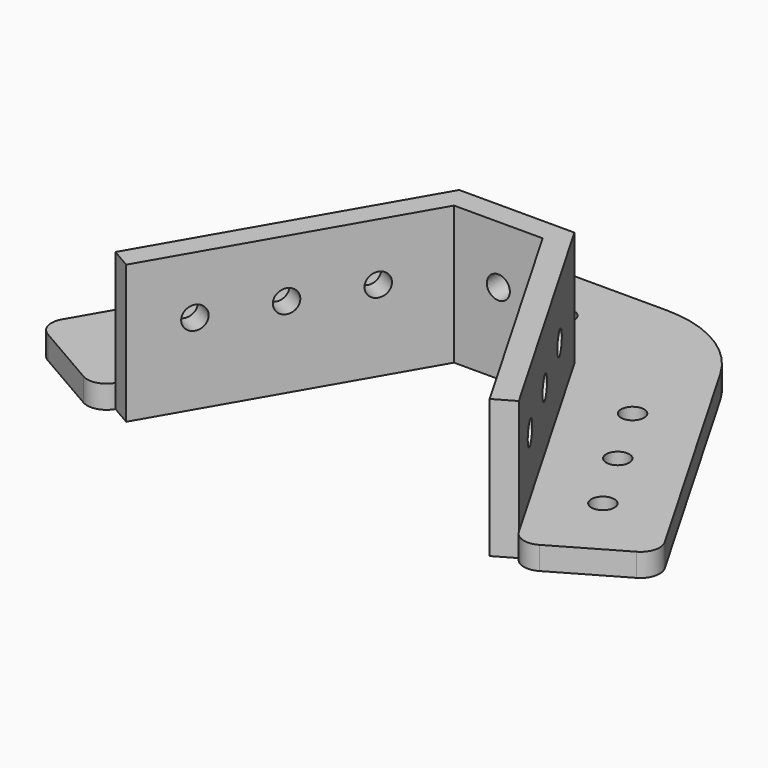
from build123d import *

# Parameters (mm, degrees)
F0_R          = 3
F1_DEPTH      = 6
F2_R          = 5
F3_R          = 5
F4_R          = 5
F5_R          = 5
F7_DEPTH      = 30
F7_DEPTH_BACK = 6
F8_R          = 3
F9_DEPTH      = 76.5570802573
F10_R         = 3
F11_DEPTH     = 36.0010005965


# Not quite as in the source:
# - a pattern or mirror of a feature is missing from the dataset's text; its kind, count and spacing are read off the source's solid


with BuildPart() as f1:
    # F0 (on Top) → F1 (new body)
    with BuildSketch(Plane.XY):
        with BuildLine():
            Line((15, 36.5101838864), (-15, 36.5101838864))
            ThreePointArc((-15, 36.5101838864), (-30, 32.490946), (-40.9807621135, 21.5101838864))
            Line((-40.9807621135, 21.5101838864), (-80.9807621135, -47.7718484163))
            Line((-80.9807621135, -47.7718484163), (-55, -62.7718484163))
            Line((-55, -62.7718484163), (-15, 6.5101838864))
            Line((-15, 6.5101838864), (15, 6.5101838864))
            Line((15, 6.5101838864), (55, -62.7718484163))
            Line((55, -62.7718484163), (80.9807621135, -47.7718484163))
            Line((80.9807621135, -47.7718484163), (40.9807621135, 21.5101838864))
            ThreePointArc((40.9807621135, 21.5101838864), (30, 32.490946), (15, 36.5101838864))
        make_face()
        with Locations((-57.9903810568, -37.9513403406)):
            Circle(F0_R, mode=Mode.SUBTRACT)
        with Locations((-47.9903810568, -20.6308322649)):
            Circle(F0_R, mode=Mode.SUBTRACT)
        with Locations((57.9903810568, -37.9513403406)):
            Circle(F0_R, mode=Mode.SUBTRACT)
        with Locations((47.9903810568, -20.6308322649)):
            Circle(F0_R, mode=Mode.SUBTRACT)
        with Locations((-37.9903810568, -3.3103241892)):
            Circle(F0_R, mode=Mode.SUBTRACT)
        with Locations((37.9903810568, -3.3103241892)):
            Circle(F0_R, mode=Mode.SUBTRACT)
        with Locations((0, 21.5101838864)):
            Circle(F0_R, mode=Mode.SUBTRACT)
    extrude(amount=F1_DEPTH)

    # F2
    f2_edges = [f1.edges().sort_by_distance(p)[0] for p in [
        (80.980762, -47.771848, 3),
    ]]
    fillet(f2_edges, radius=F2_R)

    # F3
    f3_edges = [f1.edges().sort_by_distance(p)[0] for p in [
        (55, -62.771848, 3),
    ]]
    fillet(f3_edges, radius=F3_R)

    # F4
    f4_edges = [f1.edges().sort_by_distance(p)[0] for p in [
        (-55, -62.771848, 3),
    ]]
    fillet(f4_edges, radius=F4_R)

    # F5
    f5_edges = [f1.edges().sort_by_distance(p)[0] for p in [
        (-80.980762, -47.771848, 3),
    ]]
    fillet(f5_edges, radius=F5_R)


with BuildPart() as f7:
    # F6 (on face) → F7 (new body, two sides)
    with BuildSketch(Plane.XY.offset(6)) as f7_sk:
        Polygon((52.5, -58.4417213974), (15, 6.5101838864), (-15, 6.5101838864), (-52.5, -58.4417213974), (-47.3038470608, -61.4417216956), (-11.5358980405, 0.51018329), (11.5358980405, 0.51018329), (47.3038470608, -61.4417216956), align=None)
    extrude(amount=F7_DEPTH)
    extrude(f7_sk.sketch, amount=-F7_DEPTH_BACK)

    # F8 (on face) → F9 (cut, through all)
    with BuildSketch(Plane(origin=(-8.8728393752, 5.1227362018, 0), x_dir=(0.5, 0.8660254038, 0), z_dir=(0.8660254038, -0.5, 0))):
        with Locations((-61.862015371, 21)):
            Circle(F8_R)
        with Locations((-41.862015371, 21)):
            Circle(F8_R)
        with Locations((-21.862015371, 21)):
            Circle(F8_R)
    f9 = extrude(amount=-F9_DEPTH, mode=Mode.SUBTRACT)

    # F9_copies: F9 across plane
    add(f9.mirror(Plane(origin=(0, 0, 0), x_dir=(0, 0, 1), z_dir=(1, 0, 0))), mode=Mode.SUBTRACT)

    # F10 (on face) → F11 (cut, through all)
    with BuildSketch(Plane.XZ.offset(-0.51018329)):
        with Locations((0, 21)):
            Circle(F10_R)
    extrude(amount=-F11_DEPTH, mode=Mode.SUBTRACT)


solid = Compound([f1.part, f7.part])
